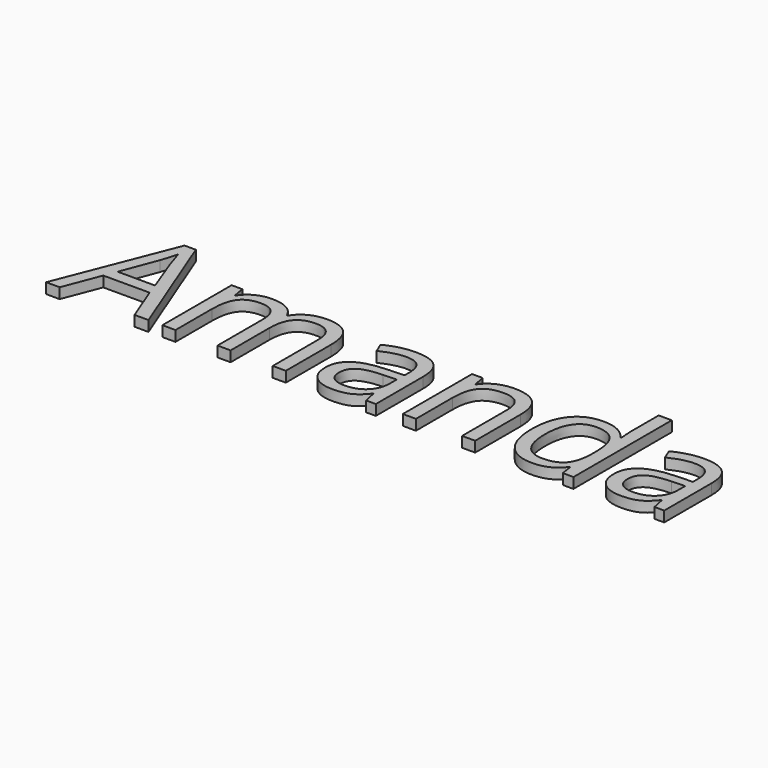
from build123d import *

# Parameters (mm, degrees)
F0_TEXT_SIZE = 39.2214894644
F1_DEPTH     = 2.54


# Not quite as in the source:
# - Text() gives the source's letters only with a copy of the font that has no kerning and outlines rounded to 1/6400 em; it was checked with that copy


with BuildPart() as f1:
    # F0 (on Top) → F1 (new body)
    with BuildSketch(Plane.XY):
        with Locations((-76.2, -8.8914562848)):
            Text('Amanda', F0_TEXT_SIZE, font='Open Sans', text_align=(TextAlign.LEFT, TextAlign.BOTTOM))
    extrude(amount=F1_DEPTH)


solid = f1.part
